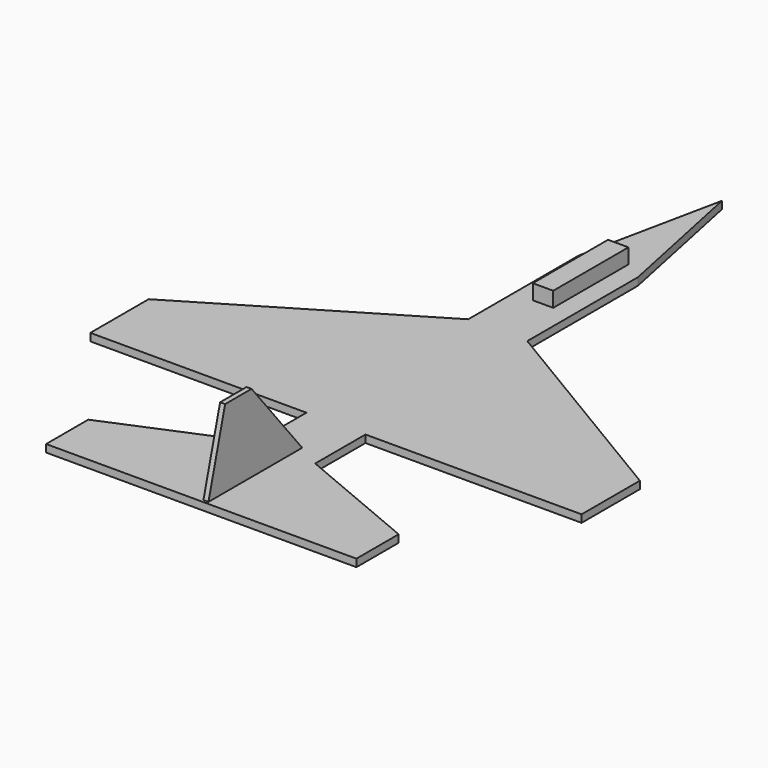
from build123d import *

# Parameters (mm, degrees)
F1_DEPTH = 1.5
F2_W     = 2.0366392564
F2_H     = 18.7370711938
F3_DEPTH = 3
F5_DEPTH = 1


# Not quite as in the source:
# - a feature names something its author has since deleted; it is built from what else it names


with BuildPart() as f1:
    # F0 (on Top) → F1 (new body)
    with BuildSketch(Plane.XY):
        Polygon((5.8843404986, 27.5437198579), (0, 55.8386333287), (-5.8843404986, 27.5437198579), (-5.8843404986, 0), (-48.9527061582, -25.7909391075), (-48.9527061582, -40.313988924), (-5.8843404986, -40.313988924), (-5.8843404986, -52.8338626027), (-30.9240873903, -63.3505582809), (-30.9240873903, -73.8672539592), (0, -73.8672539592), (30.9240873903, -73.8672539592), (30.9240873903, -63.3505582809), (5.8843404986, -52.8338626027), (5.8843404986, -40.313988924), (48.9527061582, -40.313988924), (48.9527061582, -25.7909391075), (5.8843404986, 0), align=None)
    extrude(amount=F1_DEPTH)

    # F2 (on face) → F3 (join)
    with BuildSketch(Plane.XY.offset(1.5)):
        with Locations((-1.0183196282, 20.6379326992)):
            Rectangle(F2_W, F2_H)
        with Locations((1.0183196282, 20.6379326992)):
            Rectangle(F2_W, F2_H)
    extrude(amount=F3_DEPTH)

    # F4 (on Right) → F5 (join)
    with BuildSketch(Plane.YZ):
        Polygon((-69.1700602547, 16.9719830155), (-73.7262964249, 0), (-48.7435348332, 0), (-62.592677772, 16.9719830155), align=None)
    extrude(amount=F5_DEPTH)


solid = f1.part
